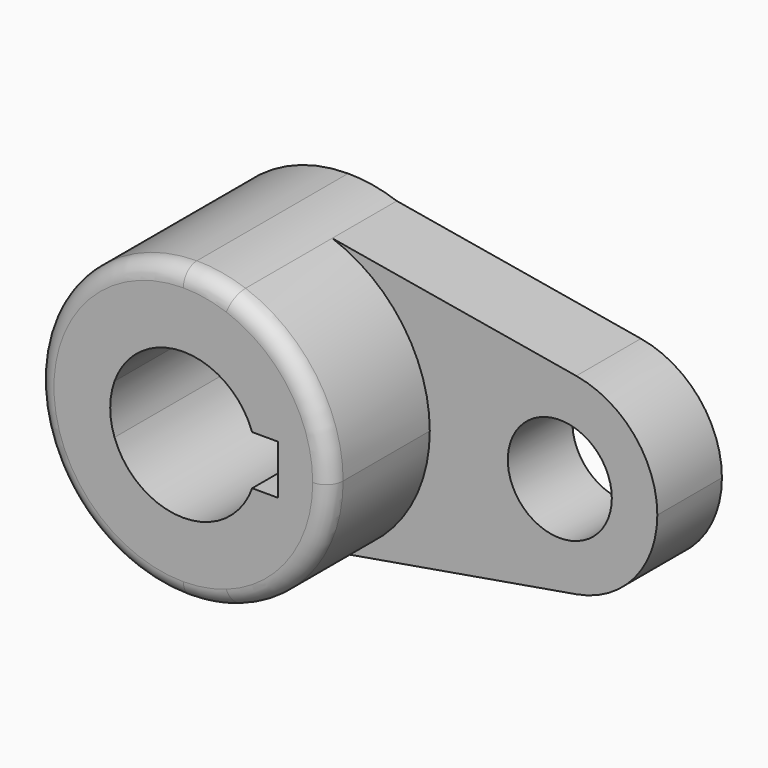
from build123d import *

# Parameters (mm, degrees)
F1_DEPTH = 40.2336
F0_R     = 10.16
F2_DEPTH = 15.7734
F3_R     = 3.302


with BuildPart() as f1:
    # F0 (on Front) → F1 (new body)
    with BuildSketch(Plane.XZ):
        with BuildLine():
            ThreePointArc((9.5121844836, 26.9452959039), (4.8253908933, 28.1646272428), (0, 28.575))
            Line((0, 28.575), (9.5121844836, 26.9452959039))
        make_face()
        with BuildLine():
            Line((9.5121844836, -26.9452959039), (0, -28.575))
            ThreePointArc((0, -28.575), (4.8253908933, -28.1646272428), (9.5121844836, -26.9452959039))
        make_face()
        with BuildLine():
            Line((9.5121844836, 26.9452959039), (0, 28.575))
            ThreePointArc((0, 28.575), (-28.575, 0), (0, -28.575))
            Line((0, -28.575), (9.5121844836, -26.9452959039))
            ThreePointArc((9.5121844836, -26.9452959039), (23.3274655355, -16.5033322905), (28.575, 0))
            ThreePointArc((28.575, 0), (23.3274655355, 16.5033322905), (9.5121844836, 26.9452959039))
        make_face()
        with BuildLine():
            ThreePointArc((-13.4477648793, 4.826), (0, 14.2875), (13.4477648793, 4.826))
            Line((13.4477648793, 4.826), (18.5293, 4.826))
            Line((18.5293, 4.826), (18.5293, -4.826))
            Line((18.5293, -4.826), (13.4477648793, -4.826))
            ThreePointArc((13.4477648793, -4.826), (0, -14.2875), (-13.4477648793, -4.826))
            Line((-13.4477648793, -4.826), (-18.5293, -4.826))
            Line((-18.5293, -4.826), (-18.5293, 4.826))
            Line((-18.5293, 4.826), (-13.4477648793, 4.826))
        make_face(mode=Mode.SUBTRACT)
        with BuildLine():
            ThreePointArc((-13.4477648793, -4.826), (-14.2875, 0), (-13.4477648793, 4.826))
            Line((-13.4477648793, 4.826), (-18.5293, 4.826))
            Line((-18.5293, 4.826), (-18.5293, -4.826))
            Line((-18.5293, -4.826), (-13.4477648793, -4.826))
        make_face()
    extrude(amount=F1_DEPTH)

    # F0 (on Front) → F2 (join)
    with BuildSketch(Plane.XZ):
        with BuildLine():
            Line((9.5121844836, 26.9452959039), (0, 28.575))
            ThreePointArc((0, 28.575), (-28.575, 0), (0, -28.575))
            Line((0, -28.575), (9.5121844836, -26.9452959039))
            ThreePointArc((9.5121844836, -26.9452959039), (23.3274655355, -16.5033322905), (28.575, 0))
            ThreePointArc((28.575, 0), (23.3274655355, 16.5033322905), (9.5121844836, 26.9452959039))
        make_face()
        with BuildLine():
            ThreePointArc((-13.4477648793, 4.826), (0, 14.2875), (13.4477648793, 4.826))
            Line((13.4477648793, 4.826), (18.5293, 4.826))
            Line((18.5293, 4.826), (18.5293, -4.826))
            Line((18.5293, -4.826), (13.4477648793, -4.826))
            ThreePointArc((13.4477648793, -4.826), (0, -14.2875), (-13.4477648793, -4.826))
            Line((-13.4477648793, -4.826), (-18.5293, -4.826))
            Line((-18.5293, -4.826), (-18.5293, 4.826))
            Line((-18.5293, 4.826), (-13.4477648793, 4.826))
        make_face(mode=Mode.SUBTRACT)
        with BuildLine():
            ThreePointArc((9.5121844836, 26.9452959039), (4.8253908933, 28.1646272428), (0, 28.575))
            Line((0, 28.575), (9.5121844836, 26.9452959039))
        make_face()
        with BuildLine():
            Line((9.5121844836, -26.9452959039), (0, -28.575))
            ThreePointArc((0, -28.575), (4.8253908933, -28.1646272428), (9.5121844836, -26.9452959039))
        make_face()
        with BuildLine():
            Line((57.1919272622, 18.7764181619), (9.5121844836, 26.9452959039))
            ThreePointArc((9.5121844836, 26.9452959039), (23.3274655355, 16.5033322905), (28.575, 0))
            ThreePointArc((28.575, 0), (23.3274655355, -16.5033322905), (9.5121844836, -26.9452959039))
            Line((9.5121844836, -26.9452959039), (57.1919272622, -18.7764181619))
            ThreePointArc((57.1919272622, -18.7764181619), (34.925, 0), (57.1919272622, 18.7764181619))
        make_face()
        with BuildLine():
            ThreePointArc((73.025, 0), (68.5383952831, 12.2804730295), (57.1919272622, 18.7764181619))
            ThreePointArc((57.1919272622, 18.7764181619), (34.925, 0), (57.1919272622, -18.7764181619))
            ThreePointArc((57.1919272622, -18.7764181619), (68.5383952831, -12.2804730295), (73.025, 0))
        make_face()
        with Locations((53.975, 0)):
            Circle(F0_R, mode=Mode.SUBTRACT)
    extrude(amount=F2_DEPTH)

    # F3
    f3_edges = [f1.edges().sort_by_distance(p)[0] for p in [
        (0, -40.2336, -28.575),
    ]]
    fillet(f3_edges, radius=F3_R)


solid = f1.part
